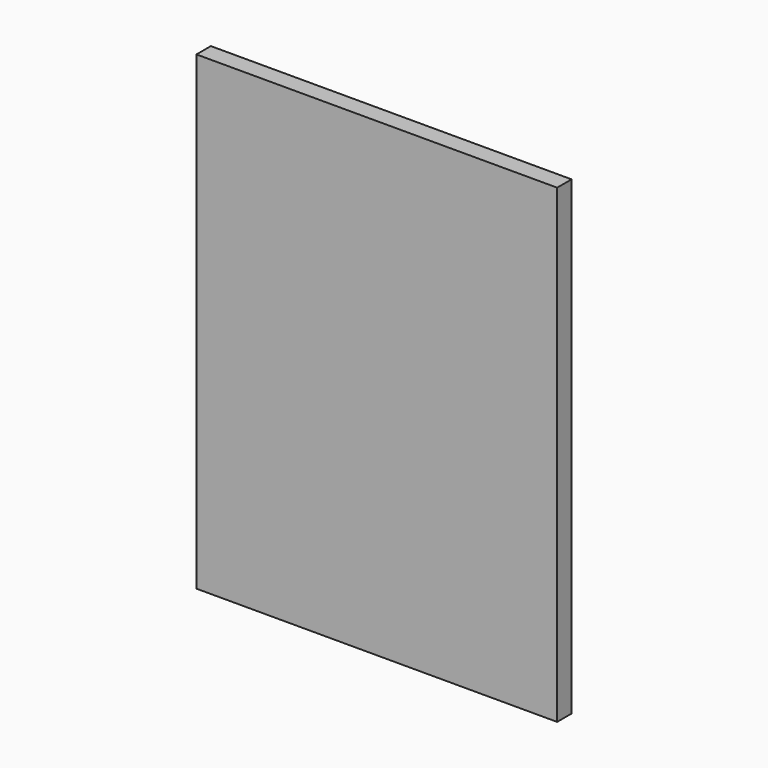
from build123d import *

# Parameters (mm, degrees)
F0_W     = 63.5
F0_H     = 82.79384
F1_DEPTH = 3.175


# Not quite as in the source:
# - a length typed as a fraction of an inch, garbled in the dataset ("3 / 203.2 mm" for 3/8 in), is restored


with BuildPart() as f1:
    # F0 (on Front) → F1 (new body)
    with BuildSketch(Plane.XZ):
        Rectangle(F0_W, F0_H)
    extrude(amount=F1_DEPTH)


solid = f1.part
